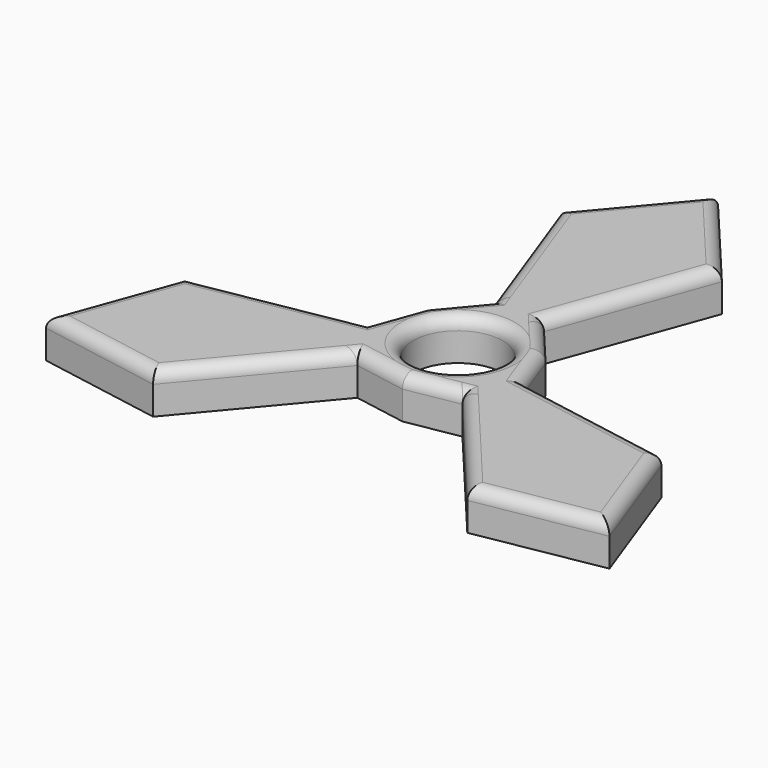
from build123d import *

# Parameters (mm, degrees)
F0_R          = 11
F1_DEPTH      = 10
F2_T1_DEPTH   = 46.1144765372
F2_T3_DEPTH   = 46.1144765372
F2_T5_DEPTH   = 46.1144765372
F2_T7_DEPTH   = 46.1144765372
F2_T9_DEPTH   = 46.1144765372
F2_T11_DEPTH  = 46.1144765372
F2_T16_DEPTH  = 33.3781970019
F2_T21_DEPTH  = 33.3781970019
F2_T26_DEPTH  = 55
F2_T31_DEPTH  = 55
F2_T36_DEPTH  = 33.3781970019
F2_T41_DEPTH  = 33.3781970019
F2_T46_DEPTH  = 55
F2_T51_DEPTH  = 55
F2_T56_DEPTH  = 33.3781970019
F2_T61_DEPTH  = 33.3781970019
F2_T66_DEPTH  = 55
F2_T71_DEPTH  = 55
F2_T79_DEPTH  = 33.3781970019
F2_T83_DEPTH  = 55
F2_T90_DEPTH  = 33.3781970019
F2_T94_DEPTH  = 55
F2_T101_DEPTH = 55
F2_T105_DEPTH = 33.3781970019
F2_T112_DEPTH = 33.3781970019
F2_T116_DEPTH = 55
F2_T123_DEPTH = 55
F2_T127_DEPTH = 33.3781970019
F2_T134_DEPTH = 33.3781970019
F2_T138_DEPTH = 55


# Not quite as in the source:
# - a fillet or chamfer that OpenCascade refuses, or shapes differently, is made with other operations: its cross-section is extruded or revolved along the edge and cut away or added


with BuildPart() as f1:
    # F0 (on Top) → F1 (new body)
    with BuildSketch(Plane.XY):
        Polygon((20, 56.1649281481), (0, 80), (-20, 56.1649281481), (-6.319194267, 18.5772233167), (-14.7578366373, 8.5204409552), (-19.2479444575, -3.8160288917), (-58.640254578, -10.7619559984), (-69.2820323028, -40), (-38.640254578, -45.4029721497), (-12.9287501905, -14.761194425), (0, -17.0408819104), (12.9287501905, -14.761194425), (38.640254578, -45.4029721497), (69.2820323028, -40), (58.640254578, -10.7619559984), (19.2479444575, -3.8160288917), (14.7578366373, 8.5204409552), (6.319194267, 18.5772233167), align=None)
        Circle(F0_R, mode=Mode.SUBTRACT)
    extrude(amount=F1_DEPTH)

    # F2: fillet of radius 3 on 19 edges, made by hand

    # F2_s2 → F2_t1 (cut)
    with BuildSketch(Plane(origin=(-14.5714030478, 17.3655219314, 0), x_dir=(0, 0, 1), z_dir=(-0.6427876097, 0.7660444431, 0))):
        with BuildLine():
            ThreePointArc((7, 51.4230087749), (9.1213203436, 50.5443291185), (10, 48.4230087749))
            Line((10, 48.4230087749), (10, 51.4230087749))
            Line((10, 51.4230087749), (7, 51.4230087749))
        make_face()
    extrude(amount=F2_T1_DEPTH, mode=Mode.SUBTRACT)

    # F2_s4 → F2_t3 (cut)
    with BuildSketch(Plane(origin=(44.2132171931, 52.6912604301, 0), x_dir=(0, 0, 1), z_dir=(-0.6427876097, -0.7660444431, 0))):
        with BuildLine():
            ThreePointArc((7, 51.4230087749), (9.1213203436, 50.5443291185), (10, 48.4230087749))
            Line((10, 48.4230087749), (10, 51.4230087749))
            Line((10, 51.4230087749), (7, 51.4230087749))
        make_face()
    extrude(amount=F2_T3_DEPTH, mode=Mode.SUBTRACT)

    # F2_s6 → F2_t5 (cut)
    with BuildSketch(Plane(origin=(-7.7532816186, -21.3019661739, 0), x_dir=(0, 0, 1), z_dir=(-0.3420201433, -0.9396926208, 0))):
        with BuildLine():
            ThreePointArc((7, 51.4230087749), (9.1213203436, 50.5443291185), (10, 48.4230087749))
            Line((10, 48.4230087749), (10, 51.4230087749))
            Line((10, 51.4230087749), (7, 51.4230087749))
        make_face()
    extrude(amount=F2_T5_DEPTH, mode=Mode.SUBTRACT)

    # F2_s8 → F2_t7 (cut)
    with BuildSketch(Plane(origin=(-67.7385786864, 11.9441390573, 0), x_dir=(0, 0, 1), z_dir=(0.984807753, -0.1736481777, 0))):
        with BuildLine():
            ThreePointArc((7, 51.4230087749), (9.1213203436, 50.5443291185), (10, 48.4230087749))
            Line((10, 48.4230087749), (10, 51.4230087749))
            Line((10, 51.4230087749), (7, 51.4230087749))
        make_face()
    extrude(amount=F2_T7_DEPTH, mode=Mode.SUBTRACT)

    # F2_s10 → F2_t9 (cut)
    with BuildSketch(Plane(origin=(22.3246846665, 3.9364442425, 0), x_dir=(0, 0, 1), z_dir=(0.984807753, 0.1736481777, 0))):
        with BuildLine():
            ThreePointArc((7, 51.4230087749), (9.1213203436, 50.5443291185), (10, 48.4230087749))
            Line((10, 48.4230087749), (10, 51.4230087749))
            Line((10, 51.4230087749), (7, 51.4230087749))
        make_face()
    extrude(amount=F2_T9_DEPTH, mode=Mode.SUBTRACT)

    # F2_s12 → F2_t11 (cut)
    with BuildSketch(Plane(origin=(23.5253614933, -64.6353994873, 0), x_dir=(0, 0, 1), z_dir=(-0.3420201433, 0.9396926208, 0))):
        with BuildLine():
            ThreePointArc((7, 51.4230087749), (9.1213203436, 50.5443291185), (10, 48.4230087749))
            Line((10, 48.4230087749), (10, 51.4230087749))
            Line((10, 51.4230087749), (7, 51.4230087749))
        make_face()
    extrude(amount=F2_T11_DEPTH, mode=Mode.SUBTRACT)


with BuildPart() as f2_tool14:
    # F2_s15 → F2_t16 (new body)
    with BuildSketch(Plane(origin=(6.043180902, -16.60350307, 0), x_dir=(0, 0, 1), z_dir=(-0.3420201433, 0.9396926208, 0))):
        with BuildLine():
            ThreePointArc((7, 16.7819926235), (9.1213203436, 15.9033129671), (10, 13.7819926235))
            Line((10, 13.7819926235), (10, 16.7819926235))
            Line((10, 16.7819926235), (7, 16.7819926235))
        make_face()
    extrude(amount=F2_T16_DEPTH)

    split(bisect_by=Plane(origin=(-0.0721828315, -0.4093691799, 0), x_dir=(0, 0, 1), z_dir=(0.1736481777, 0.984807753, 0)), keep=Keep.TOP)


with BuildPart() as f1_1:
    add(f1.part)

    # F2_t13: cut F2_tool14
    add(f2_tool14.part, mode=Mode.SUBTRACT)


with BuildPart() as f2_tool19:
    # F2_s20 → F2_t21 (new body)
    with BuildSketch(Plane(origin=(10.0976264671, -12.0338826188, 0), x_dir=(0, 0, 1), z_dir=(-0.6427876097, 0.7660444431, 0))):
        with BuildLine():
            ThreePointArc((7, 16.7819926235), (9.1213203436, 15.9033129671), (10, 13.7819926235))
            Line((10, 13.7819926235), (10, 16.7819926235))
            Line((10, 16.7819926235), (7, 16.7819926235))
        make_face()
    extrude(amount=F2_T21_DEPTH)

    split(bisect_by=Plane(origin=(-0.3906155251, 0.1421724242, 0), x_dir=(0, 0, 1), z_dir=(0.9396926208, -0.3420201433, 0)), keep=Keep.TOP)


with BuildPart() as f1_2:
    add(f1_1.part)

    # F2_t18: cut F2_tool19
    add(f2_tool19.part, mode=Mode.SUBTRACT)


with BuildPart() as f2_tool24:
    # F2_s25 → F2_t26 (new body)
    with BuildSketch(Plane(origin=(4.1446587171, 11.3873562366, 0), x_dir=(0, 0, 1), z_dir=(0.3420201433, 0.9396926208, 0))):
        with BuildLine():
            ThreePointArc((7, -0.4156843594), (9.1213203436, -1.2943640158), (10, -3.4156843594))
            Line((10, -3.4156843594), (10, -0.4156843594))
            Line((10, -0.4156843594), (7, -0.4156843594))
        make_face()
    extrude(amount=F2_T26_DEPTH)

    split(bisect_by=Plane(origin=(12.8557521937, 10.7872569243, 0), x_dir=(0, 0, 1), z_dir=(0.7660444431, 0.6427876097, 0)), keep=Keep.TOP)


with BuildPart() as f1_3:
    add(f1_2.part)

    # F2_t23: cut F2_tool24
    add(f2_tool24.part, mode=Mode.SUBTRACT)


with BuildPart() as f2_tool29:
    # F2_s30 → F2_t31 (new body)
    with BuildSketch(Plane(origin=(-22.9557666, 63.0704503798, 0), x_dir=(0, 0, 1), z_dir=(0.3420201433, -0.9396926208, 0))):
        with BuildLine():
            ThreePointArc((7, -0.4156843594), (9.1213203436, -1.2943640158), (10, -3.4156843594))
            Line((10, -3.4156843594), (10, -0.4156843594))
            Line((10, -0.4156843594), (7, -0.4156843594))
        make_face()
    extrude(amount=F2_T31_DEPTH)

    split(bisect_by=Plane(origin=(-12.8557521937, 10.7872569243, 0), x_dir=(0, 0, 1), z_dir=(-0.7660444431, 0.6427876097, 0)), keep=Keep.TOP)


with BuildPart() as f1_4:
    add(f1_3.part)

    # F2_t28: cut F2_tool29
    add(f2_tool29.part, mode=Mode.SUBTRACT)


with BuildPart() as f2_tool34:
    # F2_s35 → F2_t36 (new body)
    with BuildSketch(Plane(origin=(11.3574649994, 13.5352997158, 0), x_dir=(0, 0, 1), z_dir=(-0.6427876097, -0.7660444431, 0))):
        with BuildLine():
            ThreePointArc((7, 16.7819926235), (9.1213203436, 15.9033129671), (10, 13.7819926235))
            Line((10, 13.7819926235), (10, 16.7819926235))
            Line((10, 16.7819926235), (7, 16.7819926235))
        make_face()
    extrude(amount=F2_T36_DEPTH)

    split(bisect_by=Plane(origin=(0.3906155251, 0.1421724242, 0), x_dir=(0, 0, 1), z_dir=(-0.9396926208, -0.3420201433, 0)), keep=Keep.TOP)


with BuildPart() as f1_5:
    add(f1_4.part)

    # F2_t33: cut F2_tool34
    add(f2_tool34.part, mode=Mode.SUBTRACT)


with BuildPart() as f2_tool39:
    # F2_s40 → F2_t41 (new body)
    with BuildSketch(Plane(origin=(5.3728348205, 14.7617423478, 0), x_dir=(0, 0, 1), z_dir=(-0.3420201433, -0.9396926208, 0))):
        with BuildLine():
            ThreePointArc((7, 16.7819926235), (9.1213203436, 15.9033129671), (10, 13.7819926235))
            Line((10, 13.7819926235), (10, 16.7819926235))
            Line((10, 16.7819926235), (7, 16.7819926235))
        make_face()
    extrude(amount=F2_T41_DEPTH)

    split(bisect_by=Plane(origin=(0.0721828315, -0.4093691799, 0), x_dir=(0, 0, 1), z_dir=(-0.1736481777, 0.984807753, 0)), keep=Keep.TOP)


with BuildPart() as f1_6:
    add(f1_5.part)

    # F2_t38: cut F2_tool39
    add(f2_tool39.part, mode=Mode.SUBTRACT)


with BuildPart() as f2_tool44:
    # F2_s45 → F2_t46 (new body)
    with BuildSketch(Plane(origin=(-11.9340691414, -2.1042983793, 0), x_dir=(0, 0, 1), z_dir=(-0.984807753, -0.1736481777, 0))):
        with BuildLine():
            ThreePointArc((7, -0.4156843594), (9.1213203436, -1.2943640158), (10, -3.4156843594))
            Line((10, -3.4156843594), (10, -0.4156843594))
            Line((10, -0.4156843594), (7, -0.4156843594))
        make_face()
    extrude(amount=F2_T46_DEPTH)

    split(bisect_by=Plane(origin=(-15.7699146304, 5.7397795224, 0), x_dir=(0, 0, 1), z_dir=(-0.9396926208, 0.3420201433, 0)), keep=Keep.TOP)


with BuildPart() as f1_7:
    add(f1_6.part)

    # F2_t43: cut F2_tool44
    add(f2_tool44.part, mode=Mode.SUBTRACT)


with BuildPart() as f2_tool49:
    # F2_s50 → F2_t51 (new body)
    with BuildSketch(Plane(origin=(-43.1427289571, -51.4155022289, 0), x_dir=(0, 0, 1), z_dir=(0.6427876097, 0.7660444431, 0))):
        with BuildLine():
            ThreePointArc((7, -0.4156843594), (9.1213203436, -1.2943640158), (10, -3.4156843594))
            Line((10, -3.4156843594), (10, -0.4156843594))
            Line((10, -0.4156843594), (7, -0.4156843594))
        make_face()
    extrude(amount=F2_T51_DEPTH)

    split(bisect_by=Plane(origin=(-2.9141624367, -16.5270364467, 0), x_dir=(0, 0, 1), z_dir=(-0.1736481777, -0.984807753, 0)), keep=Keep.TOP)


with BuildPart() as f1_8:
    add(f1_7.part)

    # F2_t48: cut F2_tool49
    add(f2_tool49.part, mode=Mode.SUBTRACT)


with BuildPart() as f2_tool54:
    # F2_s55 → F2_t56 (new body)
    with BuildSketch(Plane(origin=(-17.4006459014, 3.0682033542, 0), x_dir=(0, 0, 1), z_dir=(0.984807753, -0.1736481777, 0))):
        with BuildLine():
            ThreePointArc((7, 16.7819926235), (9.1213203436, 15.9033129671), (10, 13.7819926235))
            Line((10, 13.7819926235), (10, 16.7819926235))
            Line((10, 16.7819926235), (7, 16.7819926235))
        make_face()
    extrude(amount=F2_T56_DEPTH)

    split(bisect_by=Plane(origin=(-0.3184326936, 0.2671967557, 0), x_dir=(0, 0, 1), z_dir=(0.7660444431, -0.6427876097, 0)), keep=Keep.TOP)


with BuildPart() as f1_9:
    add(f1_8.part)

    # F2_t53: cut F2_tool54
    add(f2_tool54.part, mode=Mode.SUBTRACT)


with BuildPart() as f2_tool59:
    # F2_s60 → F2_t61 (new body)
    with BuildSketch(Plane(origin=(-15.4704612876, -2.727859729, 0), x_dir=(0, 0, 1), z_dir=(0.984807753, 0.1736481777, 0))):
        with BuildLine():
            ThreePointArc((7, 16.7819926235), (9.1213203436, 15.9033129671), (10, 13.7819926235))
            Line((10, 13.7819926235), (10, 16.7819926235))
            Line((10, 16.7819926235), (7, 16.7819926235))
        make_face()
    extrude(amount=F2_T61_DEPTH)

    split(bisect_by=Plane(origin=(0.3184326936, 0.2671967557, 0), x_dir=(0, 0, 1), z_dir=(-0.7660444431, -0.6427876097, 0)), keep=Keep.TOP)


with BuildPart() as f1_10:
    add(f1_9.part)

    # F2_t58: cut F2_tool59
    add(f2_tool59.part, mode=Mode.SUBTRACT)


with BuildPart() as f2_tool64:
    # F2_s65 → F2_t66 (new body)
    with BuildSketch(Plane(origin=(7.7894104243, -9.2830578573, 0), x_dir=(0, 0, 1), z_dir=(0.6427876097, -0.7660444431, 0))):
        with BuildLine():
            ThreePointArc((7, -0.4156843594), (9.1213203436, -1.2943640158), (10, -3.4156843594))
            Line((10, -3.4156843594), (10, -0.4156843594))
            Line((10, -0.4156843594), (7, -0.4156843594))
        make_face()
    extrude(amount=F2_T66_DEPTH)

    split(bisect_by=Plane(origin=(2.9141624367, -16.5270364467, 0), x_dir=(0, 0, 1), z_dir=(0.1736481777, -0.984807753, 0)), keep=Keep.TOP)


with BuildPart() as f1_11:
    add(f1_10.part)

    # F2_t63: cut F2_tool64
    add(f2_tool64.part, mode=Mode.SUBTRACT)


with BuildPart() as f2_tool69:
    # F2_s70 → F2_t71 (new body)
    with BuildSketch(Plane(origin=(66.0984955571, -11.654948151, 0), x_dir=(0, 0, 1), z_dir=(-0.984807753, 0.1736481777, 0))):
        with BuildLine():
            ThreePointArc((7, -0.4156843594), (9.1213203436, -1.2943640158), (10, -3.4156843594))
            Line((10, -3.4156843594), (10, -0.4156843594))
            Line((10, -0.4156843594), (7, -0.4156843594))
        make_face()
    extrude(amount=F2_T71_DEPTH)

    split(bisect_by=Plane(origin=(15.7699146304, 5.7397795224, 0), x_dir=(0, 0, 1), z_dir=(0.9396926208, 0.3420201433, 0)), keep=Keep.TOP)


with BuildPart() as f1_12:
    add(f1_11.part)

    # F2_t68: cut F2_tool69
    add(f2_tool69.part, mode=Mode.SUBTRACT)

    # F2_s73 → F2_t74 (revolve, cut)
    with BuildSketch(Plane.XZ):
        with BuildLine():
            ThreePointArc((11, 7), (11.8786796564, 9.1213203436), (14, 10))
            Line((14, 10), (11, 10))
            Line((11, 10), (11, 7))
        make_face()
    revolve(axis=Axis((0, 0, 10), (0, 0, 1)), mode=Mode.SUBTRACT)


with BuildPart() as f2_tool77:
    # F2_s78 → F2_t79 (new body)
    with BuildSketch(Plane(origin=(6.043180902, -16.60350307, 0), x_dir=(0, 0, 1), z_dir=(-0.3420201433, 0.9396926208, 0))):
        with BuildLine():
            ThreePointArc((7, 16.7819926235), (9.1213203436, 15.9033129671), (10, 13.7819926235))
            Line((10, 13.7819926235), (10, 16.7819926235))
            Line((10, 16.7819926235), (7, 16.7819926235))
        make_face()
    extrude(amount=F2_T79_DEPTH)

    split(bisect_by=Plane(origin=(-0.0721828315, -0.4093691799, 0), x_dir=(0, 0, 1), z_dir=(-0.1736481777, -0.984807753, 0)), keep=Keep.TOP)


with BuildPart() as f2_tool81:
    # F2_s82 → F2_t83 (new body)
    with BuildSketch(Plane(origin=(66.0984955571, -11.654948151, 0), x_dir=(0, 0, 1), z_dir=(-0.984807753, 0.1736481777, 0))):
        with BuildLine():
            ThreePointArc((7, -0.4156843594), (9.1213203436, -1.2943640158), (10, -3.4156843594))
            Line((10, -3.4156843594), (10, -0.4156843594))
            Line((10, -0.4156843594), (7, -0.4156843594))
        make_face()
    extrude(amount=F2_T83_DEPTH)

    split(bisect_by=Plane(origin=(15.7699146304, 5.7397795224, 0), x_dir=(0, 0, 1), z_dir=(-0.9396926208, -0.3420201433, 0)), keep=Keep.TOP)


with BuildPart() as f2_tool77_1:
    add(f2_tool77.part)

    # F2_t85: intersect F2_tool81
    add(f2_tool81.part, mode=Mode.INTERSECT)


with BuildPart() as f1_13:
    add(f1_12.part)

    # F2_t75: cut F2_tool77
    add(f2_tool77_1.part, mode=Mode.SUBTRACT)


with BuildPart() as f2_tool88:
    # F2_s89 → F2_t90 (new body)
    with BuildSketch(Plane(origin=(10.0976264671, -12.0338826188, 0), x_dir=(0, 0, 1), z_dir=(-0.6427876097, 0.7660444431, 0))):
        with BuildLine():
            ThreePointArc((7, 16.7819926235), (9.1213203436, 15.9033129671), (10, 13.7819926235))
            Line((10, 13.7819926235), (10, 16.7819926235))
            Line((10, 16.7819926235), (7, 16.7819926235))
        make_face()
    extrude(amount=F2_T90_DEPTH)

    split(bisect_by=Plane(origin=(-0.3906155251, 0.1421724242, 0), x_dir=(0, 0, 1), z_dir=(-0.9396926208, 0.3420201433, 0)), keep=Keep.TOP)


with BuildPart() as f2_tool92:
    # F2_s93 → F2_t94 (new body)
    with BuildSketch(Plane(origin=(4.1446587171, 11.3873562366, 0), x_dir=(0, 0, 1), z_dir=(0.3420201433, 0.9396926208, 0))):
        with BuildLine():
            ThreePointArc((7, -0.4156843594), (9.1213203436, -1.2943640158), (10, -3.4156843594))
            Line((10, -3.4156843594), (10, -0.4156843594))
            Line((10, -0.4156843594), (7, -0.4156843594))
        make_face()
    extrude(amount=F2_T94_DEPTH)

    split(bisect_by=Plane(origin=(12.8557521937, 10.7872569243, 0), x_dir=(0, 0, 1), z_dir=(-0.7660444431, -0.6427876097, 0)), keep=Keep.TOP)


with BuildPart() as f2_tool88_1:
    add(f2_tool88.part)

    # F2_t96: intersect F2_tool92
    add(f2_tool92.part, mode=Mode.INTERSECT)


with BuildPart() as f1_14:
    add(f1_13.part)

    # F2_t86: cut F2_tool88
    add(f2_tool88_1.part, mode=Mode.SUBTRACT)


with BuildPart() as f2_tool99:
    # F2_s100 → F2_t101 (new body)
    with BuildSketch(Plane(origin=(-22.9557666, 63.0704503798, 0), x_dir=(0, 0, 1), z_dir=(0.3420201433, -0.9396926208, 0))):
        with BuildLine():
            ThreePointArc((7, -0.4156843594), (9.1213203436, -1.2943640158), (10, -3.4156843594))
            Line((10, -3.4156843594), (10, -0.4156843594))
            Line((10, -0.4156843594), (7, -0.4156843594))
        make_face()
    extrude(amount=F2_T101_DEPTH)

    split(bisect_by=Plane(origin=(-12.8557521937, 10.7872569243, 0), x_dir=(0, 0, 1), z_dir=(0.7660444431, -0.6427876097, 0)), keep=Keep.TOP)


with BuildPart() as f2_tool103:
    # F2_s104 → F2_t105 (new body)
    with BuildSketch(Plane(origin=(11.3574649994, 13.5352997158, 0), x_dir=(0, 0, 1), z_dir=(-0.6427876097, -0.7660444431, 0))):
        with BuildLine():
            ThreePointArc((7, 16.7819926235), (9.1213203436, 15.9033129671), (10, 13.7819926235))
            Line((10, 13.7819926235), (10, 16.7819926235))
            Line((10, 16.7819926235), (7, 16.7819926235))
        make_face()
    extrude(amount=F2_T105_DEPTH)

    split(bisect_by=Plane(origin=(0.3906155251, 0.1421724242, 0), x_dir=(0, 0, 1), z_dir=(0.9396926208, 0.3420201433, 0)), keep=Keep.TOP)


with BuildPart() as f2_tool99_1:
    add(f2_tool99.part)

    # F2_t107: intersect F2_tool103
    add(f2_tool103.part, mode=Mode.INTERSECT)


with BuildPart() as f1_15:
    add(f1_14.part)

    # F2_t97: cut F2_tool99
    add(f2_tool99_1.part, mode=Mode.SUBTRACT)


with BuildPart() as f2_tool110:
    # F2_s111 → F2_t112 (new body)
    with BuildSketch(Plane(origin=(5.3728348205, 14.7617423478, 0), x_dir=(0, 0, 1), z_dir=(-0.3420201433, -0.9396926208, 0))):
        with BuildLine():
            ThreePointArc((7, 16.7819926235), (9.1213203436, 15.9033129671), (10, 13.7819926235))
            Line((10, 13.7819926235), (10, 16.7819926235))
            Line((10, 16.7819926235), (7, 16.7819926235))
        make_face()
    extrude(amount=F2_T112_DEPTH)

    split(bisect_by=Plane(origin=(0.0721828315, -0.4093691799, 0), x_dir=(0, 0, 1), z_dir=(0.1736481777, -0.984807753, 0)), keep=Keep.TOP)


with BuildPart() as f2_tool114:
    # F2_s115 → F2_t116 (new body)
    with BuildSketch(Plane(origin=(-11.9340691414, -2.1042983793, 0), x_dir=(0, 0, 1), z_dir=(-0.984807753, -0.1736481777, 0))):
        with BuildLine():
            ThreePointArc((7, -0.4156843594), (9.1213203436, -1.2943640158), (10, -3.4156843594))
            Line((10, -3.4156843594), (10, -0.4156843594))
            Line((10, -0.4156843594), (7, -0.4156843594))
        make_face()
    extrude(amount=F2_T116_DEPTH)

    split(bisect_by=Plane(origin=(-15.7699146304, 5.7397795224, 0), x_dir=(0, 0, 1), z_dir=(0.9396926208, -0.3420201433, 0)), keep=Keep.TOP)


with BuildPart() as f2_tool110_1:
    add(f2_tool110.part)

    # F2_t118: intersect F2_tool114
    add(f2_tool114.part, mode=Mode.INTERSECT)


with BuildPart() as f1_16:
    add(f1_15.part)

    # F2_t108: cut F2_tool110
    add(f2_tool110_1.part, mode=Mode.SUBTRACT)


with BuildPart() as f2_tool121:
    # F2_s122 → F2_t123 (new body)
    with BuildSketch(Plane(origin=(-43.1427289571, -51.4155022289, 0), x_dir=(0, 0, 1), z_dir=(0.6427876097, 0.7660444431, 0))):
        with BuildLine():
            ThreePointArc((7, -0.4156843594), (9.1213203436, -1.2943640158), (10, -3.4156843594))
            Line((10, -3.4156843594), (10, -0.4156843594))
            Line((10, -0.4156843594), (7, -0.4156843594))
        make_face()
    extrude(amount=F2_T123_DEPTH)

    split(bisect_by=Plane(origin=(-2.9141624367, -16.5270364467, 0), x_dir=(0, 0, 1), z_dir=(0.1736481777, 0.984807753, 0)), keep=Keep.TOP)


with BuildPart() as f2_tool125:
    # F2_s126 → F2_t127 (new body)
    with BuildSketch(Plane(origin=(-17.4006459014, 3.0682033542, 0), x_dir=(0, 0, 1), z_dir=(0.984807753, -0.1736481777, 0))):
        with BuildLine():
            ThreePointArc((7, 16.7819926235), (9.1213203436, 15.9033129671), (10, 13.7819926235))
            Line((10, 13.7819926235), (10, 16.7819926235))
            Line((10, 16.7819926235), (7, 16.7819926235))
        make_face()
    extrude(amount=F2_T127_DEPTH)

    split(bisect_by=Plane(origin=(-0.3184326936, 0.2671967557, 0), x_dir=(0, 0, 1), z_dir=(-0.7660444431, 0.6427876097, 0)), keep=Keep.TOP)


with BuildPart() as f2_tool121_1:
    add(f2_tool121.part)

    # F2_t129: intersect F2_tool125
    add(f2_tool125.part, mode=Mode.INTERSECT)


with BuildPart() as f1_17:
    add(f1_16.part)

    # F2_t119: cut F2_tool121
    add(f2_tool121_1.part, mode=Mode.SUBTRACT)


with BuildPart() as f2_tool132:
    # F2_s133 → F2_t134 (new body)
    with BuildSketch(Plane(origin=(-15.4704612876, -2.727859729, 0), x_dir=(0, 0, 1), z_dir=(0.984807753, 0.1736481777, 0))):
        with BuildLine():
            ThreePointArc((7, 16.7819926235), (9.1213203436, 15.9033129671), (10, 13.7819926235))
            Line((10, 13.7819926235), (10, 16.7819926235))
            Line((10, 16.7819926235), (7, 16.7819926235))
        make_face()
    extrude(amount=F2_T134_DEPTH)

    split(bisect_by=Plane(origin=(0.3184326936, 0.2671967557, 0), x_dir=(0, 0, 1), z_dir=(0.7660444431, 0.6427876097, 0)), keep=Keep.TOP)


with BuildPart() as f2_tool136:
    # F2_s137 → F2_t138 (new body)
    with BuildSketch(Plane(origin=(7.7894104243, -9.2830578573, 0), x_dir=(0, 0, 1), z_dir=(0.6427876097, -0.7660444431, 0))):
        with BuildLine():
            ThreePointArc((7, -0.4156843594), (9.1213203436, -1.2943640158), (10, -3.4156843594))
            Line((10, -3.4156843594), (10, -0.4156843594))
            Line((10, -0.4156843594), (7, -0.4156843594))
        make_face()
    extrude(amount=F2_T138_DEPTH)

    split(bisect_by=Plane(origin=(2.9141624367, -16.5270364467, 0), x_dir=(0, 0, 1), z_dir=(-0.1736481777, 0.984807753, 0)), keep=Keep.TOP)


with BuildPart() as f2_tool132_1:
    add(f2_tool132.part)

    # F2_t140: intersect F2_tool136
    add(f2_tool136.part, mode=Mode.INTERSECT)


with BuildPart() as f1_18:
    add(f1_17.part)

    # F2_t130: cut F2_tool132
    add(f2_tool132_1.part, mode=Mode.SUBTRACT)


solid = f1_18.part
